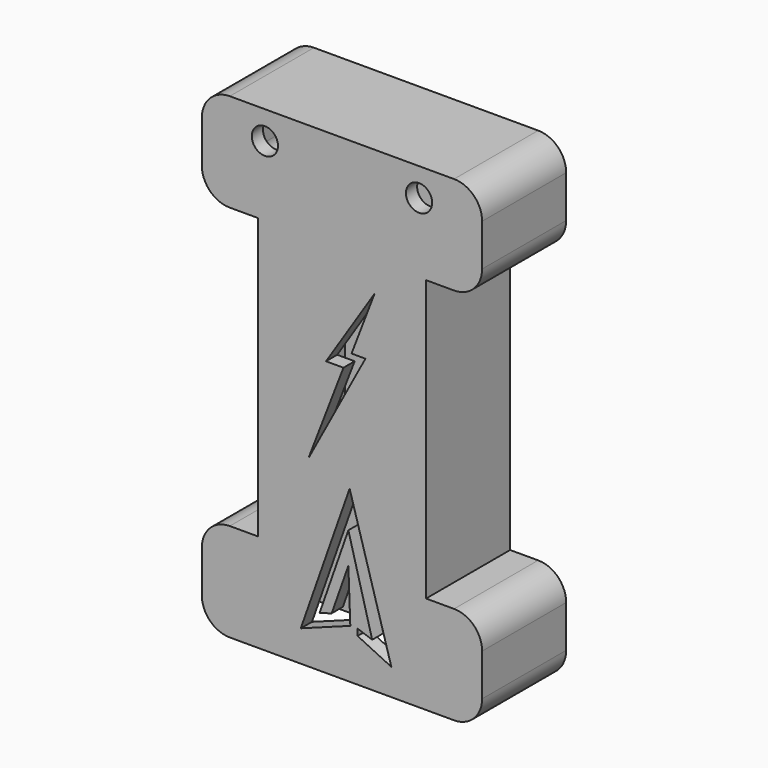
from build123d import *

# Parameters (mm, degrees)
F0_W     = 30.48
F0_H     = 50.8
F1_DEPTH = 19.05
F2_R     = 5.08
F4_T     = -2.54
F3_R     = 2.3749
F5_DEPTH = 45.59299
F7_DEPTH = 16.68371
F8_DEPTH = 25.4


# Not quite as in the source:
# - a shell that OpenCascade refuses in one call is made with other operations: the cavity is built on its own and cut out


with BuildPart() as f1:
    # F0 (on Front) → F1 (new body)
    with BuildSketch(Plane.XZ):
        with Locations((-8.951122936, -13.8477537125)):
            Rectangle(F0_W, F0_H)
        Polygon((6.288877064, -39.2477537125), (-24.191122936, -39.2477537125), (-34.351122936, -39.2477537125), (-34.351122936, -57.0277537125), (16.448877064, -57.0277537125), (16.448877064, -39.2477537125), align=None)
        Polygon((16.448877064, 29.3322462875), (-34.351122936, 29.3322462875), (-34.351122936, 11.5522462875), (-24.191122936, 11.5522462875), (6.288877064, 11.5522462875), (16.448877064, 11.5522462875), align=None)
    extrude(amount=F1_DEPTH)

    # F2
    f2_edges = [f1.edges().sort_by_distance(p)[0] for p in [
        (-34.351123, -9.525, 11.552246),
        (16.448877, -9.525, 11.552246),
        (16.448877, -9.525, 29.332246),
        (-34.351123, -9.525, 29.332246),
        (-34.351123, -9.525, -39.247754),
        (-34.351123, -9.525, -57.027754),
        (16.448877, -9.525, -57.027754),
        (16.448877, -9.525, -39.247754),
    ]]
    fillet(f2_edges, radius=F2_R)

    # F4: a shell. OpenCascade refuses it in one call, so the cavity is built on its own and cut out:
    # the body offset inwards by the wall thickness, plus a prism from it out through each open face.
    f4_core = offset(f1.part, amount=F4_T, kind=Kind.INTERSECTION, mode=Mode.PRIVATE)
    f4_exits = [f4_core.faces().sort_by_distance(p)[0] for p in [
        (-8.951123, -9.525, -54.487754),
    ]]
    add(f4_core, mode=Mode.SUBTRACT)
    extrude(f4_exits, amount=-F4_T, mode=Mode.SUBTRACT)

    # F3 (on face) → F5 (cut)
    with BuildSketch(Plane.XZ.offset(19.05)):
        with Locations((-22.921122936, 24.2522462875)):
            Circle(F3_R)
        with Locations((5.018877064, 24.2522462875)):
            Circle(F3_R)
    extrude(amount=-F5_DEPTH, mode=Mode.SUBTRACT)

    # F6 (on face) → F7 (cut)
    with BuildSketch(Plane.XZ.offset(19.05)):
        Polygon((-7.217857521, -4.5538423583), (-3.042159602, 6.352733355), (-11.8417982012, -7.2901686653), (-8.6815273389, -7.2901686653), (-15.0396805257, -23.8231290132), (-4.6957456507, -4.5538423583), align=None)
    extrude(amount=-F7_DEPTH, mode=Mode.SUBTRACT)

    # F6 (on face) → F8 (cut)
    with BuildSketch(Plane.XZ.offset(19.05)):
        Polygon((-7.217857521, -4.5538423583), (-3.042159602, 6.352733355), (-11.8417982012, -7.2901686653), (-8.6815273389, -7.2901686653), (-15.0396805257, -23.8231290132), (-4.6957456507, -4.5538423583), align=None)
        Polygon((-7.5618713163, -26.2167993933), (-16.4136328948, -51.3810502087), (-7.4369557778, -48.071410507), (-7.7901184559, -38.5827049613), (-10.809615066, -47.1666878623), (-13.0202344465, -47.8591975347), (-7.7901184559, -32.9299127667), (-3.4719579703, -49.0020355231), (-6.1175874434, -48.071410507), (-6.1175874434, -49.2577214361), (0, -52.201025188), align=None)
    extrude(amount=-F8_DEPTH, mode=Mode.SUBTRACT)


solid = f1.part
